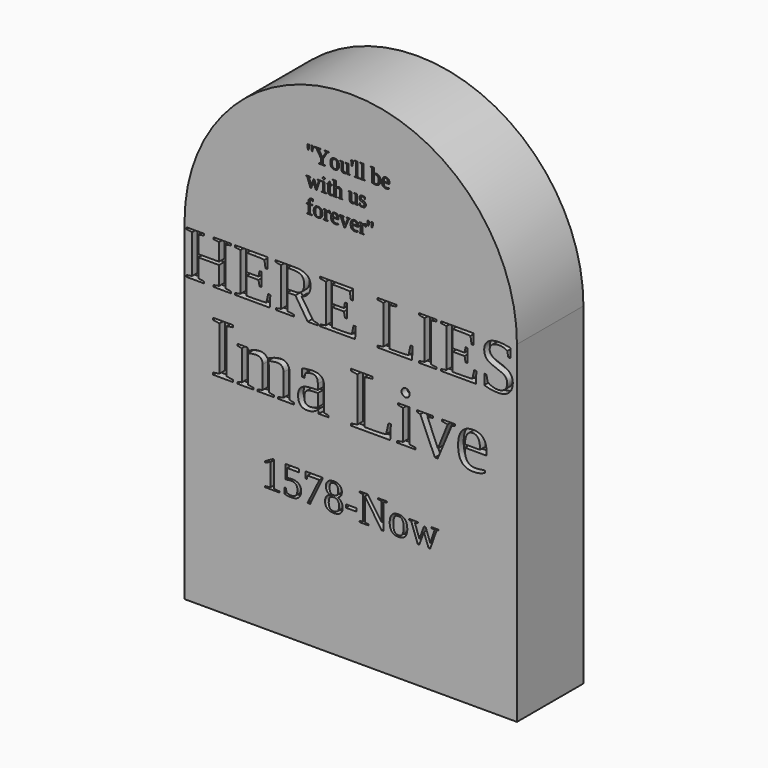
from build123d import *

# Parameters (mm, degrees)
F1_DEPTH     = 152.4
F2_TEXT_SIZE = 122.6058263411
F3_DEPTH     = 12.7
F4_TEXT_SIZE = 140.6585590707
F5_DEPTH     = 12.7
F6_TEXT_SIZE = 76.1915826135
F7_DEPTH     = 12.7
F8_TEXT_SIZE = 38.0958120028
F9_DEPTH     = 12.7


# Not quite as in the source:
# - Text() gives the source's letters only with a copy of the font that has no kerning and outlines rounded to 1/6400 em; it was checked with that copy


with BuildPart() as f1:
    # F0 (on Front) → F1 (new body)
    with BuildSketch(Plane.XZ):
        with BuildLine():
            Line((-304.8, 0), (0, 0))
            Line((0, 0), (304.8, 0))
            Line((304.8, 0), (304.8, 609.6))
            ThreePointArc((304.8, 609.6), (0, 914.4), (-304.8, 609.6))
            Line((-304.8, 609.6), (-304.8, 0))
        make_face()
    extrude(amount=F1_DEPTH)

    # F2 (on face) → F3 (cut)
    with BuildSketch(Plane.XZ.offset(152.4)):
        with Locations((-304.8, 521.3238050344)):
            Text('HERE LIES', F2_TEXT_SIZE, font='Tinos', text_align=(TextAlign.LEFT, TextAlign.BOTTOM))
    extrude(amount=-F3_DEPTH, mode=Mode.SUBTRACT)

    # F4 (on face) → F5 (cut)
    with BuildSketch(Plane.XZ.offset(152.4)):
        with Locations((-257.756809497, 379.2544007301)):
            Text('Ima Live', F4_TEXT_SIZE, font='Tinos', text_align=(TextAlign.LEFT, TextAlign.BOTTOM))
    extrude(amount=-F5_DEPTH, mode=Mode.SUBTRACT)

    # F6 (on face) → F7 (cut)
    with BuildSketch(Plane.XZ.offset(152.4)):
        with Locations((-164.2828807235, 228.6323010921)):
            Text('1578-Now', F6_TEXT_SIZE, font='Tinos', text_align=(TextAlign.LEFT, TextAlign.BOTTOM))
    extrude(amount=-F7_DEPTH, mode=Mode.SUBTRACT)

    # F8 (on face) → F9 (cut)
    with BuildSketch(Plane.XZ.offset(152.4)):
        with Locations((-82.1160413325, 783.1926345825)):
            Text('"You\'ll be', F8_TEXT_SIZE, font='Tinos', text_align=(TextAlign.LEFT, TextAlign.BOTTOM))
        with Locations((-82.1160413325, 739.3824507793)):
            Text('with us', F8_TEXT_SIZE, font='Tinos', text_align=(TextAlign.LEFT, TextAlign.BOTTOM))
        with Locations((-82.1160413325, 695.572266976)):
            Text('forever"', F8_TEXT_SIZE, font='Tinos', text_align=(TextAlign.LEFT, TextAlign.BOTTOM))
    extrude(amount=-F9_DEPTH, mode=Mode.SUBTRACT)


solid = f1.part
